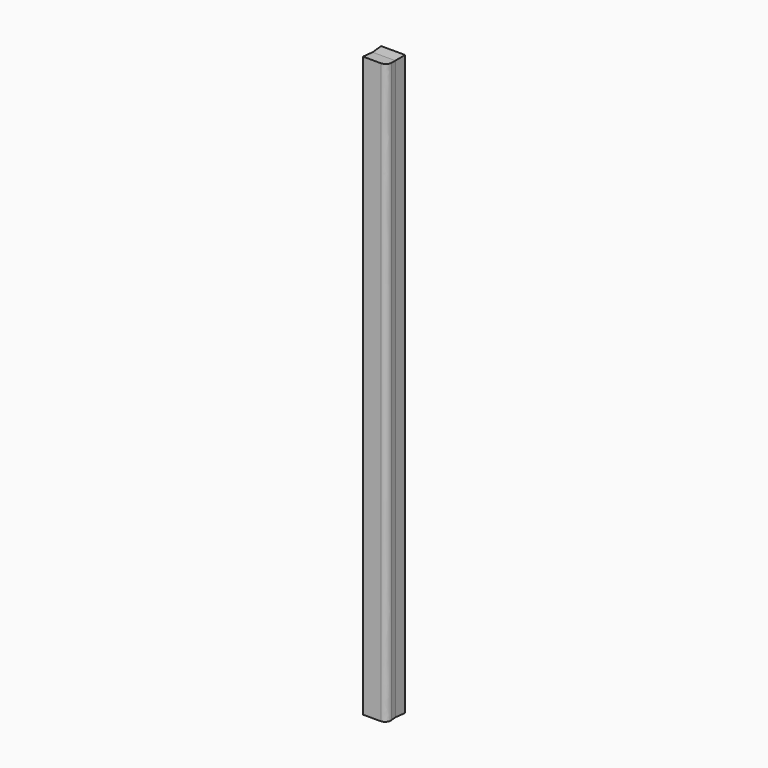
from build123d import *

# Parameters (mm, degrees)
F0_W     = 50
F0_H     = 1270
F1_DEPTH = 25
F1_TAPER = -3
F2_R     = 12.7


with BuildPart() as f1:
    # F0 (on Front) → F1 (new body, symmetric)
    with BuildSketch(Plane.XZ):
        with Locations((-25, 635)):
            Rectangle(F0_W, F0_H)
    extrude(amount=F1_DEPTH, both=True, taper=F1_TAPER)

    # F2
    f2_edges = [f1.edges().sort_by_distance(p)[0] for p in [
        (1.310194, -25, 635),
    ]]
    fillet(f2_edges, radius=F2_R)


solid = f1.part
